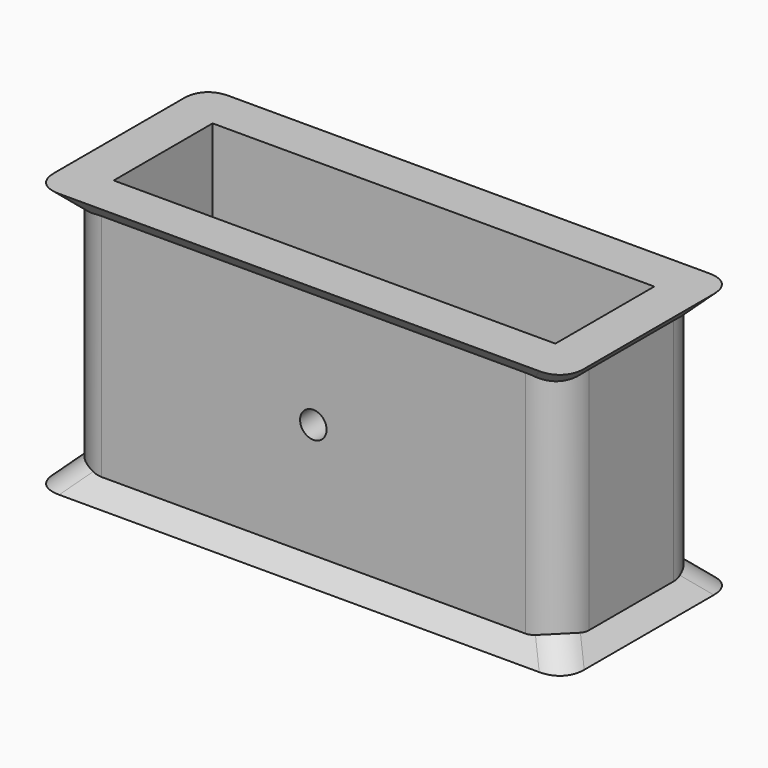
from build123d import *

# Parameters (mm, degrees)
F0_W     = 28
F0_H     = 10
F0_W_2   = 25
F0_H_2   = 7
F1_DEPTH = 15
F2_R     = 0.75
F3_DEPTH = 10.001
F6_F1_R  = 2
F6_F2_R  = 2
F6_F3_R  = 2
F6_F4_R  = 2
F6_F5_R  = 2
F6_F6_R  = 2
F6_F7_R  = 2
F6_F8_R  = 2
F6_F9_R  = 2
F6_F10_R = 2
F6_F11_R = 2
F6_F12_R = 2


# Not quite as in the source:
# - a feature of the source that left no trace in its solid (it failed there, or was rolled back) is left out
# - a pattern or mirror of a feature is missing from the dataset's text; its kind, count and spacing are read off the source's solid


with BuildPart() as f1:
    # F0 (on Top) → F1 (new body)
    with BuildSketch(Plane.XY):
        Rectangle(F0_W, F0_H)
        Rectangle(F0_W_2, F0_H_2, mode=Mode.SUBTRACT)
    extrude(amount=F1_DEPTH)

    # F2 (on face) → F3 (cut, through all)
    with BuildSketch(Plane(origin=(0, 5, 0), x_dir=(-1, 0, 0), z_dir=(0, 1, 0))):
        with Locations((0, 7.5)):
            Circle(F2_R)
    extrude(amount=-F3_DEPTH, mode=Mode.SUBTRACT)

    # F4: sweep along a path in F4_path
    with BuildLine(Plane(origin=(14, -5, 15), x_dir=(0, -1, 0), z_dir=(0, 0, -1))) as f4_path:
        Line((0, 0), (-10, 0))
        Line((-10, 0), (-10, 28))
        Line((-10, 28), (0, 28))
        Line((0, 28), (0, 0))
    # F2 (on face) → F4 (sweep)
    with BuildSketch(Plane(origin=(0, 5, 0), x_dir=(-1, 0, 0), z_dir=(0, 1, 0))):
        Polygon((-14, 14), (-14, 15), (-15, 15), align=None)
    f4 = sweep(path=f4_path.line, transition=Transition.RIGHT)

    # F4_copies: F4 across plane
    add(f4.mirror(Plane(origin=(0, 0, 7.5), x_dir=(-1, 0, 0), z_dir=(0, 0, -1))))

    # F6: fillet of radius 2 on 12 edges, made by hand

    # F6_f1
    f6_f1_edges = [f1.edges().sort_by_distance(p)[0] for p in [
        (14, 5, 7.5),
    ]]
    fillet(f6_f1_edges, radius=F6_F1_R)

    # F6_f2
    f6_f2_edges = [f1.edges().sort_by_distance(p)[0] for p in [
        (14, -5, 7.5),
    ]]
    fillet(f6_f2_edges, radius=F6_F2_R)

    # F6_f3
    f6_f3_edges = [f1.edges().sort_by_distance(p)[0] for p in [
        (14.2071067812, -5.2071067812, 0.7928932188),
    ]]
    fillet(f6_f3_edges, radius=F6_F3_R)

    # F6_f4
    f6_f4_edges = [f1.edges().sort_by_distance(p)[0] for p in [
        (14.2071067812, 5.2071067812, 0.7928932188),
    ]]
    fillet(f6_f4_edges, radius=F6_F4_R)

    # F6_f5
    f6_f5_edges = [f1.edges().sort_by_distance(p)[0] for p in [
        (-14, 5, 7.5),
    ]]
    fillet(f6_f5_edges, radius=F6_F5_R)

    # F6_f6
    f6_f6_edges = [f1.edges().sort_by_distance(p)[0] for p in [
        (14.2071067812, -5.2071067812, 14.2071067812),
    ]]
    fillet(f6_f6_edges, radius=F6_F6_R)

    # F6_f7
    f6_f7_edges = [f1.edges().sort_by_distance(p)[0] for p in [
        (14.2071067812, 5.2071067812, 14.2071067812),
    ]]
    fillet(f6_f7_edges, radius=F6_F7_R)

    # F6_f8
    f6_f8_edges = [f1.edges().sort_by_distance(p)[0] for p in [
        (-14, -5, 7.5),
    ]]
    fillet(f6_f8_edges, radius=F6_F8_R)

    # F6_f9
    f6_f9_edges = [f1.edges().sort_by_distance(p)[0] for p in [
        (-14.2071067812, -5.2071067812, 0.7928932188),
    ]]
    fillet(f6_f9_edges, radius=F6_F9_R)

    # F6_f10
    f6_f10_edges = [f1.edges().sort_by_distance(p)[0] for p in [
        (-14.2071067812, 5.2071067812, 0.7928932188),
    ]]
    fillet(f6_f10_edges, radius=F6_F10_R)

    # F6_f11
    f6_f11_edges = [f1.edges().sort_by_distance(p)[0] for p in [
        (-14.2071067812, 5.2071067812, 14.2071067812),
    ]]
    fillet(f6_f11_edges, radius=F6_F11_R)

    # F6_f12
    f6_f12_edges = [f1.edges().sort_by_distance(p)[0] for p in [
        (-14.2071067812, -5.2071067812, 14.2071067812),
    ]]
    fillet(f6_f12_edges, radius=F6_F12_R)


solid = f1.part
